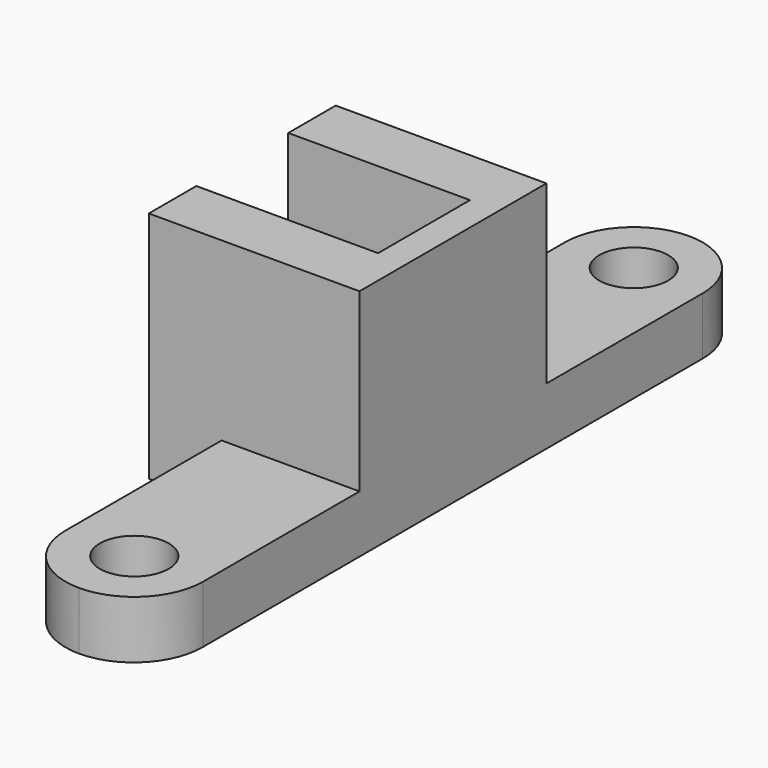
from build123d import *

# Parameters (mm, degrees)
F0_W      = 51
F0_H      = 15
F1_DEPTH  = 36
F3_R      = 9
F4_DEPTH  = 103.1
F6_DEPTH  = 15
F7_DEPTH  = 15
F2_W      = 19
F2_H      = 15.5
F8_DEPTH  = 61
F9_DEPTH  = 100
F10_DEPTH = 100
F11_DEPTH = 25
F12_DEPTH = 25


with BuildPart() as f1:
    # F0 (on Right) → F1 (new body)
    with BuildSketch(Plane.YZ):
        Polygon((30.5, 30.5), (-30.5, 30.5), (-30.5, -15.5), (-30.5, -30.5), (30.5, -30.5), (30.5, -15.5), align=None)
        with Locations((-56, -23)):
            Rectangle(F0_W, F0_H)
        with Locations((56, -23)):
            Rectangle(F0_W, F0_H)
        Polygon((-81.5, -30.5), (-81.5, -15.5), (-99.5, -15.5), (-99.5, -30.6042674929), align=None)
        Polygon((99.5, -15.5), (81.5, -15.5), (81.5, -30.5), (99.5, -30.6042674929), align=None)
    extrude(amount=F1_DEPTH)

    # F3 (on Top) → F4 (cut)
    with BuildSketch(Plane.XY):
        with Locations((18, 81.5)):
            Circle(F3_R)
        with Locations((18, -81.5)):
            Circle(F3_R)
    extrude(amount=-F4_DEPTH, mode=Mode.SUBTRACT)

    # F5 (on Front) → F6 (cut)
    with BuildSketch(Plane.XZ):
        Polygon((0, -13.7268389231), (28.6131525338, 30.7420096008), (-18.6368474662, 30.7420096008), (-18.6368474662, -30.2579903992), (-10.6368474662, -30.2579903992), align=None)
    extrude(amount=F6_DEPTH, mode=Mode.SUBTRACT)

    # F5 (on Front) → F7 (cut)
    with BuildSketch(Plane.XZ):
        Polygon((0, -13.7268389231), (28.6131525338, 30.7420096008), (-18.6368474662, 30.7420096008), (-18.6368474662, -30.2579903992), (-10.6368474662, -30.2579903992), align=None)
    extrude(amount=-F7_DEPTH, mode=Mode.SUBTRACT)

    # F2 (on face) → F8 (join)
    with BuildSketch(Plane.XY.offset(30.5)):
        with Locations((-9.5, 22.75)):
            Rectangle(F2_W, F2_H)
        with Locations((-9.5, -22.75)):
            Rectangle(F2_W, F2_H)
    extrude(amount=-F8_DEPTH)

    # F2 (on face) → F9 (cut)
    with BuildSketch(Plane.XY.offset(30.5)):
        with BuildLine():
            Line((36, -99.5), (36, -81.5))
            ThreePointArc((36, -81.5), (30.7279220614, -94.2279220614), (18, -99.5))
            Line((18, -99.5), (36, -99.5))
        make_face()
        with BuildLine():
            ThreePointArc((18, 99.5), (30.7279220614, 94.2279220614), (36, 81.5))
            Line((36, 81.5), (36, 99.5))
            Line((36, 99.5), (18, 99.5))
        make_face()
        with BuildLine():
            Line((0, 99.5), (0, 81.4999998705))
            ThreePointArc((0, 81.4999998705), (5.2720778928, 94.2279220156), (18, 99.5))
            Line((18, 99.5), (0, 99.5))
        make_face()
    extrude(amount=-F9_DEPTH, mode=Mode.SUBTRACT)

    # F2 (on face) → F10 (cut)
    with BuildSketch(Plane.XY.offset(30.5)):
        with BuildLine():
            ThreePointArc((18, -99.5), (5.2720779386, -94.2279220614), (0, -81.5))
            Line((0, -81.5), (0, -99.5))
            Line((0, -99.5), (18, -99.5))
        make_face()
        with BuildLine():
            Line((36, -99.5), (36, -81.5))
            ThreePointArc((36, -81.5), (30.7279220614, -94.2279220614), (18, -99.5))
            Line((18, -99.5), (36, -99.5))
        make_face()
    extrude(amount=-F10_DEPTH, mode=Mode.SUBTRACT)

    # F5 (on Front) → F11 (join)
    with BuildSketch(Plane.XZ):
        Polygon((0, -30.2579903992), (0, -13.7268389231), (-10.6368474662, -30.2579903992), align=None)
    extrude(amount=F11_DEPTH)

    # F5 (on Front) → F12 (join)
    with BuildSketch(Plane.XZ):
        Polygon((0, -30.2579903992), (0, -13.7268389231), (-10.6368474662, -30.2579903992), align=None)
    extrude(amount=-F12_DEPTH)


solid = f1.part
